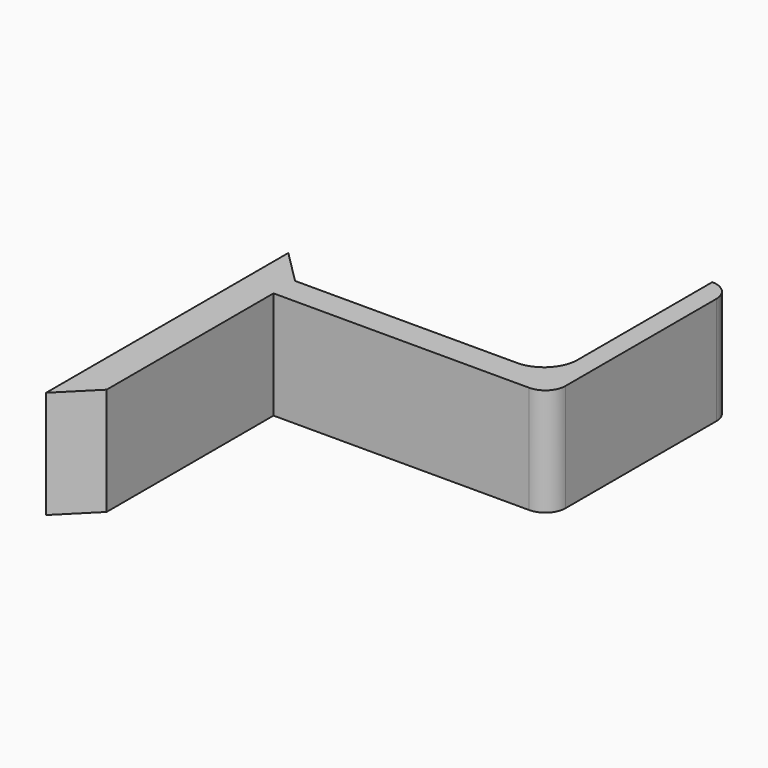
from build123d import *

# Parameters (mm, degrees)
F0_W     = 5
F0_H     = 5
F0_W_2   = 3
F0_H_2   = 30
F1_DEPTH = 16
F2_SIZE  = 4.99999
F3_SIZE  = 4.99999
F4_R     = 5
F5_R     = 2.99999


# Not quite as in the source:
# - a fillet or chamfer is up to 0.001 mm smaller than in the source, because OpenCascade refuses the exact size


with BuildPart() as f1:
    # F0 (on Top) → F1 (new body)
    with BuildSketch(Plane.XY):
        with Locations((-37.7777791023, 2.5)):
            Rectangle(F0_W, F0_H)
        Polygon((-35.2777791023, -4), (-35.2777791023, 0), (-40.2777791023, 0), (-40.2777791023, -40), (-35.2777791023, -40), align=None)
        Polygon((2.7222208977, 0), (-35.2777791023, 0), (-35.2777791023, -4), (5.7222208977, -4), (5.7222208977, 0), align=None)
        with Locations((4.2222208977, 15)):
            Rectangle(F0_W_2, F0_H_2)
    extrude(amount=F1_DEPTH)

    # F2 (size 5 in the source; OpenCascade refuses exactly that, so slightly less here)
    f2_edges = [f1.edges().sort_by_distance(p)[0] for p in [
        (-35.277779, 5, 8),
    ]]
    chamfer(f2_edges, length=F2_SIZE)

    # F3 (size 5 in the source; OpenCascade refuses exactly that, so slightly less here)
    f3_edges = [f1.edges().sort_by_distance(p)[0] for p in [
        (-35.277779, -40, 8),
    ]]
    chamfer(f3_edges, length=F3_SIZE)

    # F4
    f4_edges = [f1.edges().sort_by_distance(p)[0] for p in [
        (2.722221, 0, 8),
    ]]
    fillet(f4_edges, radius=F4_R)

    # F5 (radius 3 in the source; OpenCascade refuses exactly that, so slightly less here)
    f5_edges = [f1.edges().sort_by_distance(p)[0] for p in [
        (5.722221, -4, 8),
        (5.722221, 30, 8),
    ]]
    fillet(f5_edges, radius=F5_R)


solid = f1.part
